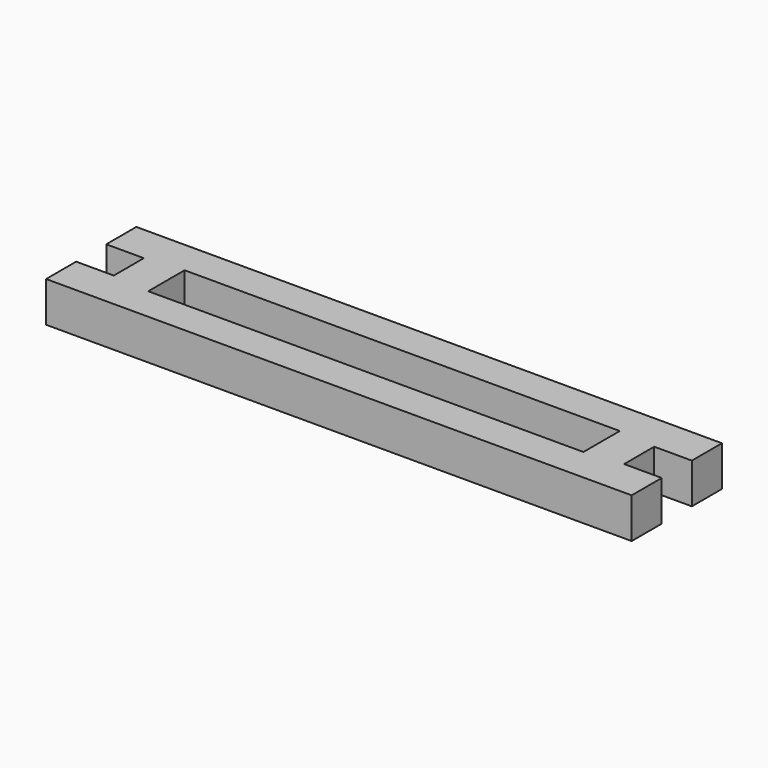
from build123d import *

# Parameters (mm, degrees)
F0_W     = 38
F0_H     = 8.4
F1_DEPTH = 3
F2_W     = 2.8
F2_H     = 3
F3_DEPTH = 2.8
F4_W     = 32.4
F4_H     = 3.3850746269
F5_DEPTH = 25


# Not quite as in the source:
# - a pattern or mirror of a feature is missing from the dataset's text; its kind, count and spacing are read off the source's solid


with BuildPart() as f1:
    # F0 (on Top) → F1 (new body)
    with BuildSketch(Plane.XY):
        Rectangle(F0_W, F0_H)
    extrude(amount=F1_DEPTH)

    # F2 (on face) → F3 (join)
    with BuildSketch(Plane(origin=(-19, 0, 0), x_dir=(0, -1, 0), z_dir=(-1, 0, 0))):
        with Locations((-2.8, 1.5)):
            Rectangle(F2_W, F2_H)
        with Locations((2.8, 1.5)):
            Rectangle(F2_W, F2_H)
    f3 = extrude(amount=F3_DEPTH)

    # F3_copies: F3 across plane
    add(f3.mirror(Plane(origin=(0, 0, 0), x_dir=(0, 0, 1), z_dir=(1, 0, 0))))

    # F4 (on face) → F5 (cut)
    with BuildSketch(Plane.XY.offset(3)):
        Rectangle(F4_W, F4_H)
    extrude(amount=-F5_DEPTH, mode=Mode.SUBTRACT)


solid = f1.part
